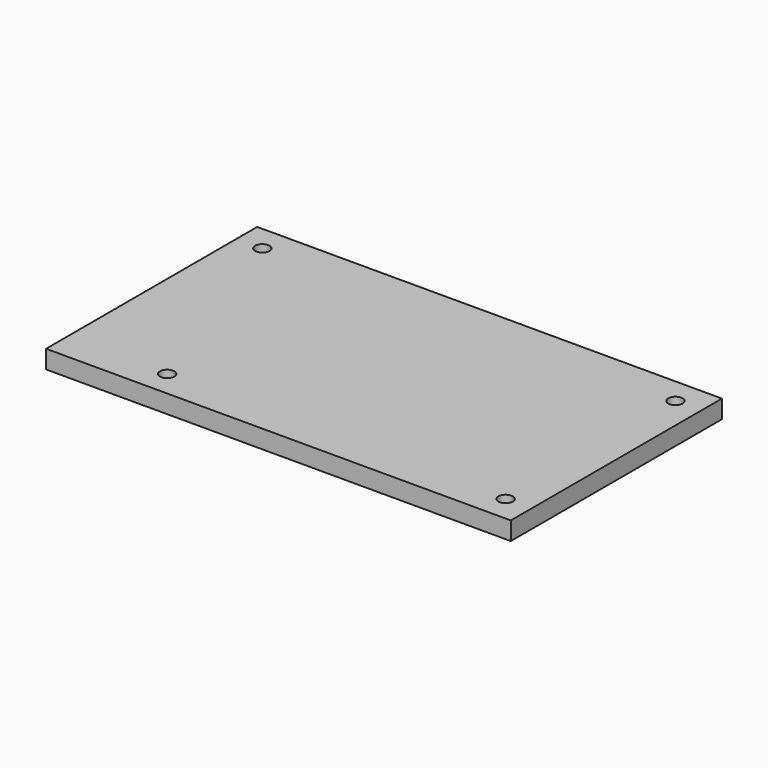
from build123d import *

# Parameters (mm, degrees)
F0_R     = 1.25
F0_W     = 68
F0_H     = 9
F1_DEPTH = 3.175


# Not quite as in the source:
# - a length typed as a fraction of an inch, garbled in the dataset ("3 / 203.2 mm" for 3/8 in), is restored
# - a feature names something its author has since deleted; it is built from what else it names


with BuildPart() as f1:
    # F0 (on Top) → F1 (new body)
    with BuildSketch(Plane.XY):
        Polygon((63.0042573512, 24.8119444549), (-17.9957426488, 24.8119444549), (-17.9957426488, 15.8119444549), (22.5042573512, 15.8119444549), (63.0042573512, 15.8119444549), align=None)
        with Locations((-13.4957426488, 20.3119444549)):
            Circle(F0_R, mode=Mode.SUBTRACT)
        with Locations((58.5042573512, 20.3119444549)):
            Circle(F0_R, mode=Mode.SUBTRACT)
        Polygon((22.5042573512, 15.8119444549), (-17.9957426488, 15.8119444549), (-17.9957426488, -21.1880555451), (-4.9957426488, -21.1880555451), (-4.9957426488, -12.1880555451), (63.0042573512, -12.1880555451), (63.0042573512, 15.8119444549), align=None)
        with Locations((29.0042573512, -16.6880555451)):
            Rectangle(F0_W, F0_H)
        with Locations((-0.4957426488, -16.6880555451)):
            Circle(F0_R, mode=Mode.SUBTRACT)
        with Locations((58.5042573512, -16.6880555451)):
            Circle(F0_R, mode=Mode.SUBTRACT)
    extrude(amount=F1_DEPTH)


solid = f1.part
